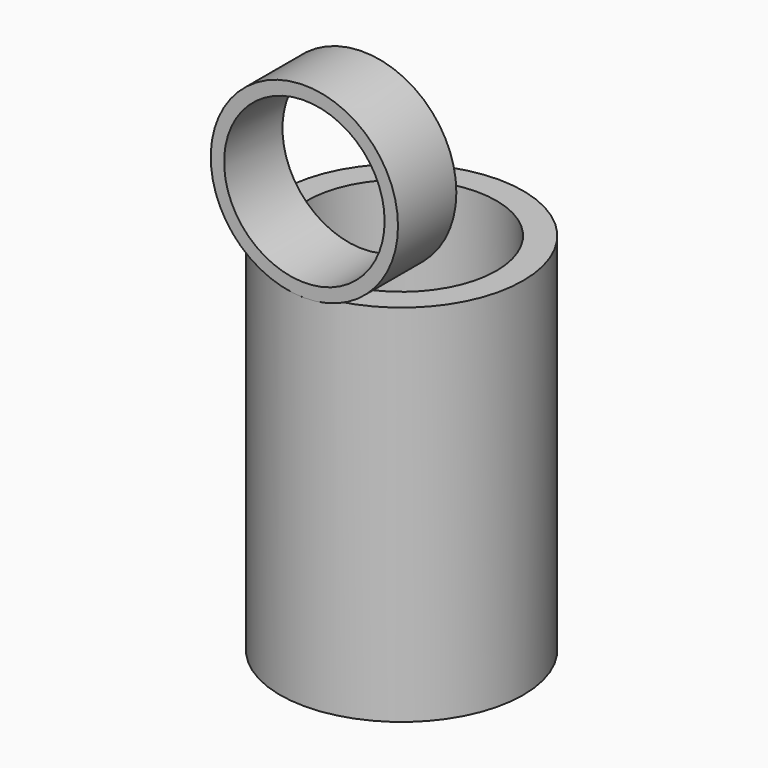
from build123d import *

# Parameters (mm, degrees)
F0_R     = 12.7
F0_R_2   = 10.922
F1_DEPTH = 19.05
F3_R     = 9.779
F3_R_2   = 8.382
F4_DEPTH = 7.62
F5_R     = 12.7
F5_R_2   = 9.906
F6_DEPTH = 19.05


with BuildPart() as f1:
    # F0 (on Top) → F1 (new body)
    with BuildSketch(Plane.XY):
        with Locations((-25.4, 25.4)):
            Circle(F0_R)
        with Locations((-25.4, 25.4)):
            Circle(F0_R_2, mode=Mode.SUBTRACT)
    extrude(amount=F1_DEPTH)



with BuildPart() as f4:
    # F3 (on offset) → F4 (new body)
    with BuildSketch(Plane.XZ.offset(-12.7)):
        with Locations((-25.4, 47.3280113715)):
            Circle(F3_R)
        with Locations((-25.4, 47.3280113715)):
            Circle(F3_R_2, mode=Mode.SUBTRACT)
    extrude(amount=-F4_DEPTH)


with BuildPart() as f1_1:
    add(f1.part)

    add(f4.part)  # F6 merges F4
    # F5 (on face) → F6 (join)
    with BuildSketch(Plane.XY.offset(19.05)):
        with Locations((-25.4, 25.4)):
            Circle(F5_R)
        with Locations((-25.4, 25.4)):
            Circle(F5_R_2, mode=Mode.SUBTRACT)
    extrude(amount=F6_DEPTH)


solid = f1_1.part
